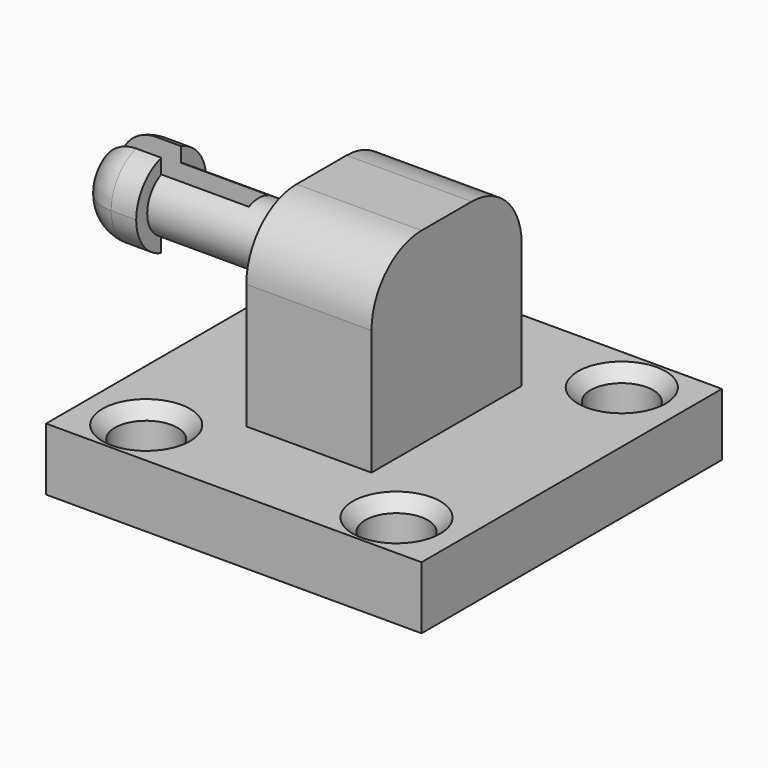
from build123d import *

# Parameters (mm, degrees)
F0_W         = 30
F0_H         = 30
F1_DEPTH     = 5
F2_W         = 5
F2_H         = 15
F3_DEPTH     = 15
F4_R         = 2.4
F5_DEPTH     = 12
F6_R         = 2.5
F7_DEPTH     = 5
F8_SIZE      = 1
F9_R         = 5
F11_DEPTH    = 5
F12_T2_ANGLE = 359.64
F12_T4_ANGLE = 359.64
F13_DEPTH    = 7


# Not quite as in the source:
# - a fillet or chamfer that OpenCascade refuses, or shapes differently, is made with other operations: its cross-section is extruded or revolved along the edge and cut away or added


with BuildPart() as f1:
    # F0 (on Top) → F1 (new body)
    with BuildSketch(Plane.XY):
        with Locations((15, 15)):
            Rectangle(F0_W, F0_H)
    extrude(amount=F1_DEPTH)

    # F2 (on face) → F3 (join)
    with BuildSketch(Plane.XY.offset(5)):
        with Locations((17.5, 15)):
            Rectangle(F2_W, F2_H)
        with Locations((12.5, 15)):
            Rectangle(F2_W, F2_H)
    extrude(amount=F3_DEPTH)

    # F4 (on face) → F5 (join)
    with BuildSketch(Plane(origin=(10, 0, 0), x_dir=(0, -1, 0), z_dir=(-1, 0, 0))):
        with Locations((-15, 14)):
            Circle(F4_R)
    extrude(amount=F5_DEPTH)

    # F6 (on face) → F7 (cut, through all)
    with BuildSketch(Plane.XY.offset(5)):
        with Locations((25, 26.25)):
            Circle(F6_R)
        with Locations((5, 26.25)):
            Circle(F6_R)
        with Locations((5, 3.75)):
            Circle(F6_R)
        with Locations((25, 3.75)):
            Circle(F6_R)
    extrude(amount=-F7_DEPTH, mode=Mode.SUBTRACT)

    # F8
    f8_edges = [f1.edges().sort_by_distance(p)[0] for p in [
        (2.5, 26.25, 5),
        (22.5, 26.25, 5),
        (22.5, 3.75, 5),
        (2.5, 3.75, 5),
    ]]
    chamfer(f8_edges, length=F8_SIZE)

    # F9
    f9_edges = [f1.edges().sort_by_distance(p)[0] for p in [
        (15, 22.5, 20),
        (15, 7.5, 20),
    ]]
    fillet(f9_edges, radius=F9_R)

    # F10 (on face) → F11 (join)
    with BuildSketch(Plane(origin=(-2, 0, 0), x_dir=(0, -1, 0), z_dir=(-1, 0, 0))):
        with BuildLine():
            Line((-16, 16.1817424229), (-16, 17.3541019662))
            ThreePointArc((-16, 17.3541019662), (-18.5, 14), (-16, 10.6458980338))
            Line((-16, 10.6458980338), (-16, 11.8182575771))
            ThreePointArc((-16, 11.8182575771), (-17.4, 14), (-16, 16.1817424229))
        make_face()
        with BuildLine():
            ThreePointArc((-14, 10.6458980338), (-12.1937569599, 11.9083499337), (-11.5, 14))
            ThreePointArc((-11.5, 14), (-12.1937569599, 16.0916500663), (-14, 17.3541019662))
            Line((-14, 17.3541019662), (-14, 16.1817424229))
            ThreePointArc((-14, 16.1817424229), (-12.9800990123, 15.2961481397), (-12.6, 14))
            ThreePointArc((-12.6, 14), (-12.9800990123, 12.7038518603), (-14, 11.8182575771))
            Line((-14, 11.8182575771), (-14, 10.6458980338))
        make_face()
        with BuildLine():
            ThreePointArc((-12.6, 14), (-12.9800990123, 15.2961481397), (-14, 16.1817424229))
            Line((-14, 16.1817424229), (-14, 11.8182575771))
            ThreePointArc((-14, 11.8182575771), (-12.9800990123, 12.7038518603), (-12.6, 14))
        make_face()
        with BuildLine():
            Line((-16, 11.8182575771), (-16, 16.1817424229))
            ThreePointArc((-16, 16.1817424229), (-17.4, 14), (-16, 11.8182575771))
        make_face()
    extrude(amount=F11_DEPTH)

    # F12: fillet of radius 3 on 2 edges, made by hand

    # F12_s1 → F12_t2 (revolve, cut)
    with BuildSketch(Plane(origin=(0, 0.0441300513, 14.0469854057), x_dir=(1, 0, 0), z_dir=(0, -0.0031415875, -0.9999950652))):
        with BuildLine():
            ThreePointArc((-4, -11.4559437532), (-6.1213203436, -12.3346234097), (-7, -14.4559437532))
            Line((-7, -14.4559437532), (-7, -11.4559437532))
            Line((-7, -11.4559437532), (-4, -11.4559437532))
        make_face()
    revolve(axis=Axis((-7, 15, 14), (-1, 0, 0)), revolution_arc=F12_T2_ANGLE, mode=Mode.SUBTRACT)

    # F12_s3 → F12_t4 (revolve, cut)
    with BuildSketch(Plane(origin=(0, 0.0441300513, 14.0469854057), x_dir=(1, 0, 0), z_dir=(0, 0.0031415875, 0.9999950652))):
        with BuildLine():
            ThreePointArc((-4, 18.4559437532), (-6.1213203436, 17.5772640968), (-7, 15.4559437532))
            Line((-7, 15.4559437532), (-7, 18.4559437532))
            Line((-7, 18.4559437532), (-4, 18.4559437532))
        make_face()
    revolve(axis=Axis((-7, 15, 14), (-1, 0, 0)), revolution_arc=F12_T4_ANGLE, mode=Mode.SUBTRACT)

    # F13 (cut): a face of the model
    f13_faces = [f1.faces().sort_by_distance(p)[0] for p in [
        (-2, 15, 14),
    ]]
    extrude(f13_faces, amount=-F13_DEPTH, mode=Mode.SUBTRACT)


solid = f1.part
